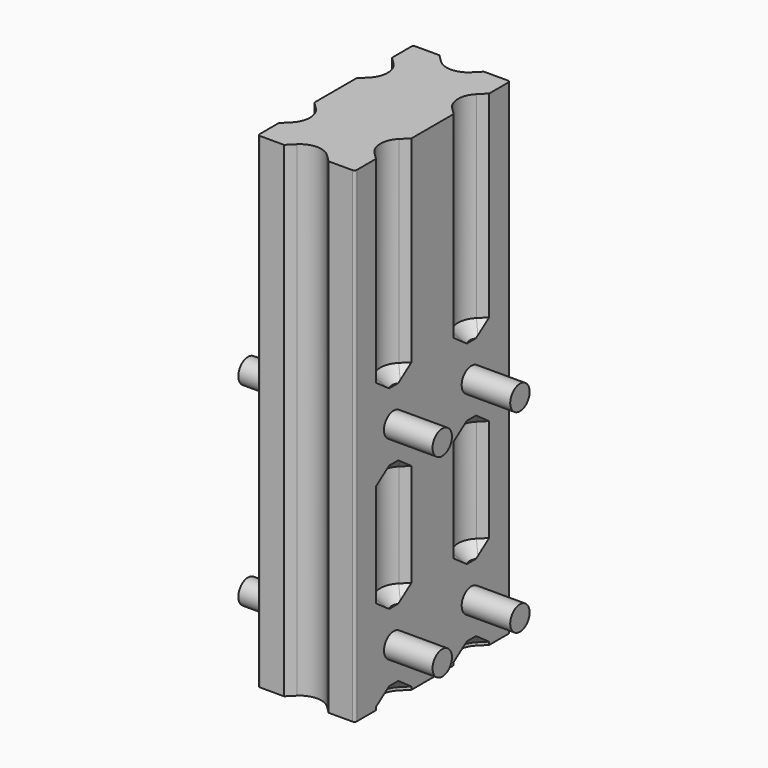
from build123d import *

# Parameters (mm, degrees)
F1_DEPTH      = 100
F2_W          = 14
F2_H          = 14
F2_R          = 2.5
F3_DEPTH      = 10
F4_DEPTH      = 20
F5_T4_ANGLE   = 90
F5_T9_ANGLE   = 90
F5_T14_ANGLE  = 90
F5_T19_ANGLE  = 90
F5_T24_ANGLE  = 90
F5_T29_ANGLE  = 90
F5_T34_ANGLE  = 90
F5_T39_ANGLE  = 90
F5_T44_ANGLE  = 90
F5_T49_ANGLE  = 90
F5_T54_ANGLE  = 90
F5_T59_ANGLE  = 90
F5_T64_ANGLE  = 90
F5_T69_ANGLE  = 90
F5_T74_ANGLE  = 90
F5_T79_ANGLE  = 90
F5_T84_DEPTH  = 8.2297199044
F5_T89_DEPTH  = 8.2297199044
F5_T94_DEPTH  = 8.2297199044
F5_T99_DEPTH  = 8.2297199044
F5_T104_DEPTH = 8.2297199044
F5_T109_DEPTH = 8.2297199044
F5_T114_DEPTH = 8.2297199044
F5_T119_DEPTH = 8.2297199044
F5_T124_DEPTH = 8.2297199044
F5_T129_DEPTH = 8.2297199044
F5_T134_DEPTH = 8.2297199044
F5_T139_DEPTH = 8.2297199044
F5_T144_DEPTH = 8.2297199044
F5_T149_DEPTH = 8.2297199044
F5_T154_DEPTH = 8.2297199044
F5_T159_DEPTH = 8.2297199044
F5_T164_DEPTH = 8.2297199044
F5_T169_DEPTH = 8.2297199044
F5_T174_DEPTH = 8.2297199044
F5_T179_DEPTH = 8.2297199044
F5_T184_DEPTH = 8.2297199044
F5_T189_DEPTH = 8.2297199044
F5_T194_DEPTH = 8.2297199044
F5_T199_DEPTH = 8.2297199044
F5_T204_DEPTH = 8.2297199044
F5_T209_DEPTH = 8.2297199044
F5_T214_DEPTH = 8.2297199044
F5_T219_DEPTH = 8.2297199044
F5_T224_DEPTH = 8.2297199044
F5_T229_DEPTH = 8.2297199044
F5_T234_DEPTH = 8.2297199044
F5_T239_DEPTH = 8.2297199044


# Not quite as in the source:
# - a fillet or chamfer that OpenCascade refuses, or shapes differently, is made with other operations: its cross-section is extruded or revolved along the edge and cut away or added


with BuildPart() as f1:
    # F0 (on Top) → F1 (new body)
    with BuildSketch(Plane.XY):
        with BuildLine():
            Line((-10, 5.42), (-10, 0))
            Line((-10, 0), (-10, -5.42))
            Line((-10, -5.42), (-8.545, -6.875))
            Line((-8.545, -6.875), (-8.2, -6.875))
            Line((-8.2, -6.875), (-6.2, -6.875))
            Line((-6.2, -6.875), (-6.2, -13.125))
            Line((-6.2, -13.125), (-8.2, -13.125))
            Line((-8.2, -13.125), (-8.545, -13.125))
            Line((-8.545, -13.125), (-10, -14.58))
            Line((-10, -14.58), (-10, -19.5))
            ThreePointArc((-10, -19.5), (-9.8535533906, -19.8535533906), (-9.5, -20))
            Line((-9.5, -20), (-4.58, -20))
            Line((-4.58, -20), (-3.125, -18.545))
            Line((-3.125, -18.545), (-3.125, -18.2))
            Line((-3.125, -18.2), (-3.125, -16.2))
            Line((-3.125, -16.2), (0, -16.2))
            Line((0, -16.2), (3.125, -16.2))
            Line((3.125, -16.2), (3.125, -18.2))
            Line((3.125, -18.2), (3.125, -18.545))
            Line((3.125, -18.545), (4.58, -20))
            Line((4.58, -20), (9.5, -20))
            ThreePointArc((9.5, -20), (9.8535533906, -19.8535533906), (10, -19.5))
            Line((10, -19.5), (10, -14.58))
            Line((10, -14.58), (8.545, -13.125))
            Line((8.545, -13.125), (8.2, -13.125))
            Line((8.2, -13.125), (6.2, -13.125))
            Line((6.2, -13.125), (6.2, -6.875))
            Line((6.2, -6.875), (8.2, -6.875))
            Line((8.2, -6.875), (8.545, -6.875))
            Line((8.545, -6.875), (10, -5.42))
            Line((10, -5.42), (10, 0))
            Line((10, 0), (10, 5.42))
            Line((10, 5.42), (8.545, 6.875))
            Line((8.545, 6.875), (8.2, 6.875))
            Line((8.2, 6.875), (6.2, 6.875))
            Line((6.2, 6.875), (6.2, 13.125))
            Line((6.2, 13.125), (8.2, 13.125))
            Line((8.2, 13.125), (8.545, 13.125))
            Line((8.545, 13.125), (10, 14.58))
            Line((10, 14.58), (10, 19.5))
            ThreePointArc((10, 19.5), (9.8535533906, 19.8535533906), (9.5, 20))
            Line((9.5, 20), (4.58, 20))
            Line((4.58, 20), (3.125, 18.545))
            Line((3.125, 18.545), (3.125, 18.2))
            Line((3.125, 18.2), (3.125, 16.2))
            Line((3.125, 16.2), (0, 16.2))
            Line((0, 16.2), (-3.125, 16.2))
            Line((-3.125, 16.2), (-3.125, 18.2))
            Line((-3.125, 18.2), (-3.125, 18.545))
            Line((-3.125, 18.545), (-4.58, 20))
            Line((-4.58, 20), (-9.5, 20))
            ThreePointArc((-9.5, 20), (-9.8535533906, 19.8535533906), (-10, 19.5))
            Line((-10, 19.5), (-10, 14.58))
            Line((-10, 14.58), (-8.545, 13.125))
            Line((-8.545, 13.125), (-8.2, 13.125))
            Line((-8.2, 13.125), (-6.2, 13.125))
            Line((-6.2, 13.125), (-6.2, 6.875))
            Line((-6.2, 6.875), (-8.2, 6.875))
            Line((-8.2, 6.875), (-8.545, 6.875))
            Line((-8.545, 6.875), (-10, 5.42))
        make_face()
        with BuildLine():
            ThreePointArc((8.545, 6.875), (7.2505826176, 10), (8.545, 13.125))
            Line((8.545, 13.125), (8.2, 13.125))
            Line((8.2, 13.125), (6.2, 13.125))
            Line((6.2, 13.125), (6.2, 6.875))
            Line((6.2, 6.875), (8.2, 6.875))
            Line((8.2, 6.875), (8.545, 6.875))
        make_face()
        with BuildLine():
            Line((8.2, -13.125), (8.545, -13.125))
            ThreePointArc((8.545, -13.125), (7.2505826176, -10), (8.545, -6.875))
            Line((8.545, -6.875), (8.2, -6.875))
            Line((8.2, -6.875), (6.2, -6.875))
            Line((6.2, -6.875), (6.2, -13.125))
            Line((6.2, -13.125), (8.2, -13.125))
        make_face()
        with BuildLine():
            Line((-3.125, -18.2), (-3.125, -18.545))
            ThreePointArc((-3.125, -18.545), (0, -17.2505826176), (3.125, -18.545))
            Line((3.125, -18.545), (3.125, -18.2))
            Line((3.125, -18.2), (3.125, -16.2))
            Line((3.125, -16.2), (0, -16.2))
            Line((0, -16.2), (-3.125, -16.2))
            Line((-3.125, -16.2), (-3.125, -18.2))
        make_face()
        with BuildLine():
            Line((-8.2, -6.875), (-8.545, -6.875))
            ThreePointArc((-8.545, -6.875), (-7.2505826176, -10), (-8.545, -13.125))
            Line((-8.545, -13.125), (-8.2, -13.125))
            Line((-8.2, -13.125), (-6.2, -13.125))
            Line((-6.2, -13.125), (-6.2, -6.875))
            Line((-6.2, -6.875), (-8.2, -6.875))
        make_face()
        with BuildLine():
            ThreePointArc((-8.545, 13.125), (-7.2505826176, 10), (-8.545, 6.875))
            Line((-8.545, 6.875), (-8.2, 6.875))
            Line((-8.2, 6.875), (-6.2, 6.875))
            Line((-6.2, 6.875), (-6.2, 13.125))
            Line((-6.2, 13.125), (-8.2, 13.125))
            Line((-8.2, 13.125), (-8.545, 13.125))
        make_face()
        with BuildLine():
            ThreePointArc((3.125, 18.545), (0, 17.2505826176), (-3.125, 18.545))
            Line((-3.125, 18.545), (-3.125, 18.2))
            Line((-3.125, 18.2), (-3.125, 16.2))
            Line((-3.125, 16.2), (0, 16.2))
            Line((0, 16.2), (3.125, 16.2))
            Line((3.125, 16.2), (3.125, 18.2))
            Line((3.125, 18.2), (3.125, 18.545))
        make_face()
    extrude(amount=F1_DEPTH)

    # F2 (on Right) → F3 (join, symmetric)
    with BuildSketch(Plane.YZ):
        with Locations((10, 50)):
            Rectangle(F2_W, F2_H)
        with Locations((10, 50)):
            Circle(F2_R, mode=Mode.SUBTRACT)
        with Locations((-10, 50)):
            Rectangle(F2_W, F2_H)
        with Locations((-10, 50)):
            Circle(F2_R, mode=Mode.SUBTRACT)
        with Locations((-10, 10)):
            Rectangle(F2_W, F2_H)
        with Locations((-10, 10)):
            Circle(F2_R, mode=Mode.SUBTRACT)
        with Locations((10, 10)):
            Rectangle(F2_W, F2_H)
        with Locations((10, 10)):
            Circle(F2_R, mode=Mode.SUBTRACT)
    extrude(amount=F3_DEPTH, both=True)

    # F2 (on Right) → F4 (join, symmetric)
    with BuildSketch(Plane.YZ):
        with Locations((10, 10)):
            Circle(F2_R)
        with Locations((10, 50)):
            Circle(F2_R)
        with Locations((-10, 10)):
            Circle(F2_R)
        with Locations((-10, 50)):
            Circle(F2_R)
    extrude(amount=F4_DEPTH, both=True)

    # F5: chamfer of 2.4 on 48 edges, made by hand


with BuildPart() as f5_tool2:
    # F5_s3 → F5_t4 (revolve)
    with BuildSketch(Plane(origin=(-10.835, 10.835, 0), x_dir=(0, 0, 1), z_dir=(-0.7071067812, 0.7071067812, 0))):
        Polygon((43, 0.8385490578), (40.6, 3.2385490578), (43, 3.2385490578), align=None)
    revolve(axis=Axis((-11.67, 10, 43), (0, 0, -1)), revolution_arc=F5_T4_ANGLE)

    split(bisect_by=Plane.YZ.offset(-10), keep=Keep.TOP)


with BuildPart() as f1_1:
    add(f1.part)

    # F5_t1: union F5_tool2
    add(f5_tool2.part)


with BuildPart() as f5_tool7:
    # F5_s8 → F5_t9 (revolve)
    with BuildSketch(Plane(origin=(-10.835, 10.835, 0), x_dir=(0, 0, 1), z_dir=(-0.7071067812, 0.7071067812, 0))):
        Polygon((17, 0.8385490578), (19.4, 3.2385490578), (17, 3.2385490578), align=None)
    revolve(axis=Axis((-11.67, 10, 17), (0, 0, -1)), revolution_arc=F5_T9_ANGLE)

    split(bisect_by=Plane.YZ.offset(-10), keep=Keep.TOP)


with BuildPart() as f1_2:
    add(f1_1.part)

    # F5_t6: union F5_tool7
    add(f5_tool7.part)


with BuildPart() as f5_tool12:
    # F5_s13 → F5_t14 (revolve)
    with BuildSketch(Plane(origin=(-10.835, 10.835, 0), x_dir=(0, 0, 1), z_dir=(-0.7071067812, 0.7071067812, 0))):
        Polygon((57, 0.8385490578), (59.4, 3.2385490578), (57, 3.2385490578), align=None)
    revolve(axis=Axis((-11.67, 10, 57), (0, 0, -1)), revolution_arc=F5_T14_ANGLE)

    split(bisect_by=Plane.YZ.offset(-10), keep=Keep.TOP)


with BuildPart() as f1_3:
    add(f1_2.part)

    # F5_t11: union F5_tool12
    add(f5_tool12.part)


with BuildPart() as f5_tool17:
    # F5_s18 → F5_t19 (revolve)
    with BuildSketch(Plane(origin=(-0.835, 0.835, 0), x_dir=(0, 0, 1), z_dir=(-0.7071067812, 0.7071067812, 0))):
        Polygon((57, -13.3035865659), (59.4, -10.9035865659), (57, -10.9035865659), align=None)
    revolve(axis=Axis((-11.67, -10, 57), (0, 0, -1)), revolution_arc=F5_T19_ANGLE)

    split(bisect_by=Plane.YZ.offset(-10), keep=Keep.TOP)


with BuildPart() as f1_4:
    add(f1_3.part)

    # F5_t16: union F5_tool17
    add(f5_tool17.part)


with BuildPart() as f5_tool22:
    # F5_s23 → F5_t24 (revolve)
    with BuildSketch(Plane(origin=(-0.835, 0.835, 0), x_dir=(0, 0, 1), z_dir=(-0.7071067812, 0.7071067812, 0))):
        Polygon((17, -13.3035865659), (19.4, -10.9035865659), (17, -10.9035865659), align=None)
    revolve(axis=Axis((-11.67, -10, 17), (0, 0, -1)), revolution_arc=F5_T24_ANGLE)

    split(bisect_by=Plane.YZ.offset(-10), keep=Keep.TOP)


with BuildPart() as f1_5:
    add(f1_4.part)

    # F5_t21: union F5_tool22
    add(f5_tool22.part)


with BuildPart() as f5_tool27:
    # F5_s28 → F5_t29 (revolve)
    with BuildSketch(Plane(origin=(-0.835, 0.835, 0), x_dir=(0, 0, 1), z_dir=(-0.7071067812, 0.7071067812, 0))):
        Polygon((43, -13.3035865659), (40.6, -10.9035865659), (43, -10.9035865659), align=None)
    revolve(axis=Axis((-11.67, -10, 43), (0, 0, -1)), revolution_arc=F5_T29_ANGLE)

    split(bisect_by=Plane.YZ.offset(-10), keep=Keep.TOP)


with BuildPart() as f1_6:
    add(f1_5.part)

    # F5_t26: union F5_tool27
    add(f5_tool27.part)


with BuildPart() as f5_tool32:
    # F5_s33 → F5_t34 (revolve)
    with BuildSketch(Plane(origin=(-0.835, 0.835, 0), x_dir=(0, 0, 1), z_dir=(-0.7071067812, 0.7071067812, 0))):
        Polygon((0.6, -10.9035865659), (3, -13.3035865659), (3, -10.9035865659), align=None)
    revolve(axis=Axis((-11.67, -10, 3), (0, 0, -1)), revolution_arc=F5_T34_ANGLE)

    split(bisect_by=Plane.YZ.offset(-10), keep=Keep.TOP)


with BuildPart() as f1_7:
    add(f1_6.part)

    # F5_t31: union F5_tool32
    add(f5_tool32.part)


with BuildPart() as f5_tool37:
    # F5_s38 → F5_t39 (revolve)
    with BuildSketch(Plane(origin=(-10.835, 10.835, 0), x_dir=(0, 0, 1), z_dir=(-0.7071067812, 0.7071067812, 0))):
        Polygon((3, 0.8385490578), (0.6, 3.2385490578), (3, 3.2385490578), align=None)
    revolve(axis=Axis((-11.67, 10, 3), (0, 0, -1)), revolution_arc=F5_T39_ANGLE)

    split(bisect_by=Plane.YZ.offset(-10), keep=Keep.TOP)


with BuildPart() as f1_8:
    add(f1_7.part)

    # F5_t36: union F5_tool37
    add(f5_tool37.part)


with BuildPart() as f5_tool42:
    # F5_s43 → F5_t44 (revolve)
    with BuildSketch(Plane(origin=(10.835, -10.835, 0), x_dir=(0, 0, 1), z_dir=(0.7071067812, -0.7071067812, 0))):
        Polygon((57, 0.8385490578), (59.4, 3.2385490578), (57, 3.2385490578), align=None)
    revolve(axis=Axis((11.67, -10, 57), (0, 0, -1)), revolution_arc=F5_T44_ANGLE)

    split(bisect_by=Plane.YZ.offset(10), keep=Keep.BOTTOM)


with BuildPart() as f1_9:
    add(f1_8.part)

    # F5_t41: union F5_tool42
    add(f5_tool42.part)


with BuildPart() as f5_tool47:
    # F5_s48 → F5_t49 (revolve)
    with BuildSketch(Plane(origin=(10.835, -10.835, 0), x_dir=(0, 0, 1), z_dir=(0.7071067812, -0.7071067812, 0))):
        Polygon((17, 0.8385490578), (19.4, 3.2385490578), (17, 3.2385490578), align=None)
    revolve(axis=Axis((11.67, -10, 17), (0, 0, -1)), revolution_arc=F5_T49_ANGLE)

    split(bisect_by=Plane.YZ.offset(10), keep=Keep.BOTTOM)


with BuildPart() as f1_10:
    add(f1_9.part)

    # F5_t46: union F5_tool47
    add(f5_tool47.part)


with BuildPart() as f5_tool52:
    # F5_s53 → F5_t54 (revolve)
    with BuildSketch(Plane(origin=(0.835, -0.835, 0), x_dir=(0, 0, 1), z_dir=(0.7071067812, -0.7071067812, 0))):
        Polygon((17, -13.3035865659), (19.4, -10.9035865659), (17, -10.9035865659), align=None)
    revolve(axis=Axis((11.67, 10, 17), (0, 0, -1)), revolution_arc=F5_T54_ANGLE)

    split(bisect_by=Plane.YZ.offset(10), keep=Keep.BOTTOM)


with BuildPart() as f1_11:
    add(f1_10.part)

    # F5_t51: union F5_tool52
    add(f5_tool52.part)


with BuildPart() as f5_tool57:
    # F5_s58 → F5_t59 (revolve)
    with BuildSketch(Plane(origin=(0.835, -0.835, 0), x_dir=(0, 0, 1), z_dir=(0.7071067812, -0.7071067812, 0))):
        Polygon((57, -13.3035865659), (59.4, -10.9035865659), (57, -10.9035865659), align=None)
    revolve(axis=Axis((11.67, 10, 57), (0, 0, -1)), revolution_arc=F5_T59_ANGLE)

    split(bisect_by=Plane.YZ.offset(10), keep=Keep.BOTTOM)


with BuildPart() as f1_12:
    add(f1_11.part)

    # F5_t56: union F5_tool57
    add(f5_tool57.part)


with BuildPart() as f5_tool62:
    # F5_s63 → F5_t64 (revolve)
    with BuildSketch(Plane(origin=(0.835, -0.835, 0), x_dir=(0, 0, 1), z_dir=(0.7071067812, -0.7071067812, 0))):
        Polygon((43, -13.3035865659), (40.6, -10.9035865659), (43, -10.9035865659), align=None)
    revolve(axis=Axis((11.67, 10, 43), (0, 0, -1)), revolution_arc=F5_T64_ANGLE)

    split(bisect_by=Plane.YZ.offset(10), keep=Keep.BOTTOM)


with BuildPart() as f1_13:
    add(f1_12.part)

    # F5_t61: union F5_tool62
    add(f5_tool62.part)


with BuildPart() as f5_tool67:
    # F5_s68 → F5_t69 (revolve)
    with BuildSketch(Plane(origin=(10.835, -10.835, 0), x_dir=(0, 0, 1), z_dir=(0.7071067812, -0.7071067812, 0))):
        Polygon((43, 0.8385490578), (40.6, 3.2385490578), (43, 3.2385490578), align=None)
    revolve(axis=Axis((11.67, -10, 43), (0, 0, -1)), revolution_arc=F5_T69_ANGLE)

    split(bisect_by=Plane.YZ.offset(10), keep=Keep.BOTTOM)


with BuildPart() as f1_14:
    add(f1_13.part)

    # F5_t66: union F5_tool67
    add(f5_tool67.part)


with BuildPart() as f5_tool72:
    # F5_s73 → F5_t74 (revolve)
    with BuildSketch(Plane(origin=(10.835, -10.835, 0), x_dir=(0, 0, 1), z_dir=(0.7071067812, -0.7071067812, 0))):
        Polygon((0.6, 3.2385490578), (3, 0.8385490578), (3, 3.2385490578), align=None)
    revolve(axis=Axis((11.67, -10, 3), (0, 0, -1)), revolution_arc=F5_T74_ANGLE)

    split(bisect_by=Plane.YZ.offset(10), keep=Keep.BOTTOM)


with BuildPart() as f1_15:
    add(f1_14.part)

    # F5_t71: union F5_tool72
    add(f5_tool72.part)


with BuildPart() as f5_tool77:
    # F5_s78 → F5_t79 (revolve)
    with BuildSketch(Plane(origin=(0.835, -0.835, 0), x_dir=(0, 0, 1), z_dir=(0.7071067812, -0.7071067812, 0))):
        Polygon((0.6, -10.9035865659), (3, -13.3035865659), (3, -10.9035865659), align=None)
    revolve(axis=Axis((11.67, 10, 3), (0, 0, -1)), revolution_arc=F5_T79_ANGLE)

    split(bisect_by=Plane.YZ.offset(10), keep=Keep.BOTTOM)


with BuildPart() as f1_16:
    add(f1_15.part)

    # F5_t76: union F5_tool77
    add(f5_tool77.part)


with BuildPart() as f5_tool82:
    # F5_s83 → F5_t84 (new body)
    with BuildSketch(Plane(origin=(-6.6542907516, -6.6542907516, 0), x_dir=(0, 0, 1), z_dir=(0.7071067812, 0.7071067812, 0))):
        Polygon((0.6, -10.9035865659), (3, -13.3035865659), (3, -10.9035865659), align=None)
    extrude(amount=F5_T84_DEPTH)

    split(bisect_by=Plane.YZ.offset(-10), keep=Keep.TOP)


with BuildPart() as f1_17:
    add(f1_16.part)

    # F5_t81: union F5_tool82
    add(f5_tool82.part)


with BuildPart() as f5_tool87:
    # F5_s88 → F5_t89 (new body)
    with BuildSketch(Plane(origin=(-10.835, 10.835, 0), x_dir=(0, 0, 1), z_dir=(-0.7071067812, 0.7071067812, 0))):
        Polygon((3, 0.8385490578), (0.6, 3.2385490578), (3, 3.2385490578), align=None)
    extrude(amount=F5_T89_DEPTH)

    split(bisect_by=Plane.YZ.offset(-10), keep=Keep.TOP)


with BuildPart() as f1_18:
    add(f1_17.part)

    # F5_t86: union F5_tool87
    add(f5_tool87.part)


with BuildPart() as f5_tool92:
    # F5_s93 → F5_t94 (new body)
    with BuildSketch(Plane(origin=(-0.835, 0.835, 0), x_dir=(0, 0, 1), z_dir=(-0.7071067812, 0.7071067812, 0))):
        Polygon((0.6, -10.9035865659), (3, -13.3035865659), (3, -10.9035865659), align=None)
    extrude(amount=F5_T94_DEPTH)

    split(bisect_by=Plane.YZ.offset(-10), keep=Keep.TOP)


with BuildPart() as f1_19:
    add(f1_18.part)

    # F5_t91: union F5_tool92
    add(f5_tool92.part)


with BuildPart() as f5_tool97:
    # F5_s98 → F5_t99 (new body)
    with BuildSketch(Plane(origin=(-16.6542907516, -16.6542907516, 0), x_dir=(0, 0, 1), z_dir=(0.7071067812, 0.7071067812, 0))):
        Polygon((0.6, 3.2385490578), (3, 0.8385490578), (3, 3.2385490578), align=None)
    extrude(amount=F5_T99_DEPTH)

    split(bisect_by=Plane.YZ.offset(-10), keep=Keep.TOP)


with BuildPart() as f1_20:
    add(f1_19.part)

    # F5_t96: union F5_tool97
    add(f5_tool97.part)


with BuildPart() as f5_tool102:
    # F5_s103 → F5_t104 (new body)
    with BuildSketch(Plane(origin=(10.835, -10.835, 0), x_dir=(0, 0, 1), z_dir=(0.7071067812, -0.7071067812, 0))):
        Polygon((0.6, 3.2385490578), (3, 0.8385490578), (3, 3.2385490578), align=None)
    extrude(amount=F5_T104_DEPTH)

    split(bisect_by=Plane.YZ.offset(10), keep=Keep.BOTTOM)


with BuildPart() as f1_21:
    add(f1_20.part)

    # F5_t101: union F5_tool102
    add(f5_tool102.part)


with BuildPart() as f5_tool107:
    # F5_s108 → F5_t109 (new body)
    with BuildSketch(Plane(origin=(6.6542907516, 6.6542907516, 0), x_dir=(0, 0, 1), z_dir=(-0.7071067812, -0.7071067812, 0))):
        Polygon((0.6, -10.9035865659), (3, -13.3035865659), (3, -10.9035865659), align=None)
    extrude(amount=F5_T109_DEPTH)

    split(bisect_by=Plane.YZ.offset(10), keep=Keep.BOTTOM)


with BuildPart() as f1_22:
    add(f1_21.part)

    # F5_t106: union F5_tool107
    add(f5_tool107.part)


with BuildPart() as f5_tool112:
    # F5_s113 → F5_t114 (new body)
    with BuildSketch(Plane(origin=(0.835, -0.835, 0), x_dir=(0, 0, 1), z_dir=(0.7071067812, -0.7071067812, 0))):
        Polygon((0.6, -10.9035865659), (3, -13.3035865659), (3, -10.9035865659), align=None)
    extrude(amount=F5_T114_DEPTH)

    split(bisect_by=Plane.YZ.offset(10), keep=Keep.BOTTOM)


with BuildPart() as f1_23:
    add(f1_22.part)

    # F5_t111: union F5_tool112
    add(f5_tool112.part)


with BuildPart() as f5_tool117:
    # F5_s118 → F5_t119 (new body)
    with BuildSketch(Plane(origin=(16.6542907516, 16.6542907516, 0), x_dir=(0, 0, 1), z_dir=(-0.7071067812, -0.7071067812, 0))):
        Polygon((0.6, 3.2385490578), (3, 0.8385490578), (3, 3.2385490578), align=None)
    extrude(amount=F5_T119_DEPTH)

    split(bisect_by=Plane.YZ.offset(10), keep=Keep.BOTTOM)


with BuildPart() as f1_24:
    add(f1_23.part)

    # F5_t116: union F5_tool117
    add(f5_tool117.part)


with BuildPart() as f5_tool122:
    # F5_s123 → F5_t124 (new body)
    with BuildSketch(Plane(origin=(-16.6542907516, 16.6542907516, 0), x_dir=(0, 0, 1), z_dir=(0.7071067812, -0.7071067812, 0))):
        Polygon((59.4, -3.2385490578), (57, -0.8385490578), (57, -3.2385490578), align=None)
    extrude(amount=F5_T124_DEPTH)

    split(bisect_by=Plane.YZ.offset(-10), keep=Keep.TOP)


with BuildPart() as f1_25:
    add(f1_24.part)

    # F5_t121: union F5_tool122
    add(f5_tool122.part)


with BuildPart() as f5_tool127:
    # F5_s128 → F5_t129 (new body)
    with BuildSketch(Plane(origin=(-0.835, -0.835, 0), x_dir=(0, 0, 1), z_dir=(-0.7071067812, -0.7071067812, 0))):
        Polygon((57, 13.3035865659), (59.4, 10.9035865659), (57, 10.9035865659), align=None)
    extrude(amount=F5_T129_DEPTH)

    split(bisect_by=Plane.YZ.offset(-10), keep=Keep.TOP)


with BuildPart() as f1_26:
    add(f1_25.part)

    # F5_t126: union F5_tool127
    add(f5_tool127.part)


with BuildPart() as f5_tool132:
    # F5_s133 → F5_t134 (new body)
    with BuildSketch(Plane(origin=(-6.6542907516, 6.6542907516, 0), x_dir=(0, 0, 1), z_dir=(0.7071067812, -0.7071067812, 0))):
        Polygon((59.4, 10.9035865659), (57, 13.3035865659), (57, 10.9035865659), align=None)
    extrude(amount=F5_T134_DEPTH)

    split(bisect_by=Plane.YZ.offset(-10), keep=Keep.TOP)


with BuildPart() as f1_27:
    add(f1_26.part)

    # F5_t131: union F5_tool132
    add(f5_tool132.part)


with BuildPart() as f5_tool137:
    # F5_s138 → F5_t139 (new body)
    with BuildSketch(Plane(origin=(-10.835, -10.835, 0), x_dir=(0, 0, 1), z_dir=(-0.7071067812, -0.7071067812, 0))):
        Polygon((57, -0.8385490578), (59.4, -3.2385490578), (57, -3.2385490578), align=None)
    extrude(amount=F5_T139_DEPTH)

    split(bisect_by=Plane.YZ.offset(-10), keep=Keep.TOP)


with BuildPart() as f1_28:
    add(f1_27.part)

    # F5_t136: union F5_tool137
    add(f5_tool137.part)


with BuildPart() as f5_tool142:
    # F5_s143 → F5_t144 (new body)
    with BuildSketch(Plane(origin=(-6.6542907516, 6.6542907516, 0), x_dir=(0, 0, 1), z_dir=(0.7071067812, -0.7071067812, 0))):
        Polygon((19.4, 10.9035865659), (17, 13.3035865659), (17, 10.9035865659), align=None)
    extrude(amount=F5_T144_DEPTH)

    split(bisect_by=Plane.YZ.offset(-10), keep=Keep.TOP)


with BuildPart() as f1_29:
    add(f1_28.part)

    # F5_t141: union F5_tool142
    add(f5_tool142.part)


with BuildPart() as f5_tool147:
    # F5_s148 → F5_t149 (new body)
    with BuildSketch(Plane(origin=(-0.835, 0.835, 0), x_dir=(0, 0, 1), z_dir=(-0.7071067812, 0.7071067812, 0))):
        Polygon((40.6, -10.9035865659), (43, -13.3035865659), (43, -10.9035865659), align=None)
    extrude(amount=F5_T149_DEPTH)

    split(bisect_by=Plane.YZ.offset(-10), keep=Keep.TOP)


with BuildPart() as f1_30:
    add(f1_29.part)

    # F5_t146: union F5_tool147
    add(f5_tool147.part)


with BuildPart() as f5_tool152:
    # F5_s153 → F5_t154 (new body)
    with BuildSketch(Plane(origin=(-10.835, -10.835, 0), x_dir=(0, 0, 1), z_dir=(-0.7071067812, -0.7071067812, 0))):
        Polygon((17, -0.8385490578), (19.4, -3.2385490578), (17, -3.2385490578), align=None)
    extrude(amount=F5_T154_DEPTH)

    split(bisect_by=Plane.YZ.offset(-10), keep=Keep.TOP)


with BuildPart() as f1_31:
    add(f1_30.part)

    # F5_t151: union F5_tool152
    add(f5_tool152.part)


with BuildPart() as f5_tool157:
    # F5_s158 → F5_t159 (new body)
    with BuildSketch(Plane(origin=(-16.6542907516, -16.6542907516, 0), x_dir=(0, 0, 1), z_dir=(0.7071067812, 0.7071067812, 0))):
        Polygon((40.6, 3.2385490578), (43, 0.8385490578), (43, 3.2385490578), align=None)
    extrude(amount=F5_T159_DEPTH)

    split(bisect_by=Plane.YZ.offset(-10), keep=Keep.TOP)


with BuildPart() as f1_32:
    add(f1_31.part)

    # F5_t156: union F5_tool157
    add(f5_tool157.part)


with BuildPart() as f5_tool162:
    # F5_s163 → F5_t164 (new body)
    with BuildSketch(Plane(origin=(-0.835, -0.835, 0), x_dir=(0, 0, 1), z_dir=(-0.7071067812, -0.7071067812, 0))):
        Polygon((19.4, 10.9035865659), (17, 13.3035865659), (17, 10.9035865659), align=None)
    extrude(amount=F5_T164_DEPTH)

    split(bisect_by=Plane.YZ.offset(-10), keep=Keep.TOP)


with BuildPart() as f1_33:
    add(f1_32.part)

    # F5_t161: union F5_tool162
    add(f5_tool162.part)


with BuildPart() as f5_tool167:
    # F5_s168 → F5_t169 (new body)
    with BuildSketch(Plane(origin=(-6.6542907516, -6.6542907516, 0), x_dir=(0, 0, 1), z_dir=(0.7071067812, 0.7071067812, 0))):
        Polygon((40.6, -10.9035865659), (43, -13.3035865659), (43, -10.9035865659), align=None)
    extrude(amount=F5_T169_DEPTH)

    split(bisect_by=Plane.YZ.offset(-10), keep=Keep.TOP)


with BuildPart() as f1_34:
    add(f1_33.part)

    # F5_t166: union F5_tool167
    add(f5_tool167.part)


with BuildPart() as f5_tool172:
    # F5_s173 → F5_t174 (new body)
    with BuildSketch(Plane(origin=(-10.835, 10.835, 0), x_dir=(0, 0, 1), z_dir=(-0.7071067812, 0.7071067812, 0))):
        Polygon((43, 0.8385490578), (40.6, 3.2385490578), (43, 3.2385490578), align=None)
    extrude(amount=F5_T174_DEPTH)

    split(bisect_by=Plane.YZ.offset(-10), keep=Keep.TOP)


with BuildPart() as f1_35:
    add(f1_34.part)

    # F5_t171: union F5_tool172
    add(f5_tool172.part)


with BuildPart() as f5_tool177:
    # F5_s178 → F5_t179 (new body)
    with BuildSketch(Plane(origin=(-16.6542907516, 16.6542907516, 0), x_dir=(0, 0, 1), z_dir=(0.7071067812, -0.7071067812, 0))):
        Polygon((19.4, -3.2385490578), (17, -0.8385490578), (17, -3.2385490578), align=None)
    extrude(amount=F5_T179_DEPTH)

    split(bisect_by=Plane.YZ.offset(-10), keep=Keep.TOP)


with BuildPart() as f1_36:
    add(f1_35.part)

    # F5_t176: union F5_tool177
    add(f5_tool177.part)


with BuildPart() as f5_tool182:
    # F5_s183 → F5_t184 (new body)
    with BuildSketch(Plane(origin=(16.6542907516, -16.6542907516, 0), x_dir=(0, 0, 1), z_dir=(-0.7071067812, 0.7071067812, 0))):
        Polygon((59.4, -3.2385490578), (57, -0.8385490578), (57, -3.2385490578), align=None)
    extrude(amount=F5_T184_DEPTH)

    split(bisect_by=Plane.YZ.offset(10), keep=Keep.BOTTOM)


with BuildPart() as f1_37:
    add(f1_36.part)

    # F5_t181: union F5_tool182
    add(f5_tool182.part)


with BuildPart() as f5_tool187:
    # F5_s188 → F5_t189 (new body)
    with BuildSketch(Plane(origin=(0.835, 0.835, 0), x_dir=(0, 0, 1), z_dir=(0.7071067812, 0.7071067812, 0))):
        Polygon((57, 13.3035865659), (59.4, 10.9035865659), (57, 10.9035865659), align=None)
    extrude(amount=F5_T189_DEPTH)

    split(bisect_by=Plane.YZ.offset(10), keep=Keep.BOTTOM)


with BuildPart() as f1_38:
    add(f1_37.part)

    # F5_t186: union F5_tool187
    add(f5_tool187.part)


with BuildPart() as f5_tool192:
    # F5_s193 → F5_t194 (new body)
    with BuildSketch(Plane(origin=(6.6542907516, -6.6542907516, 0), x_dir=(0, 0, 1), z_dir=(-0.7071067812, 0.7071067812, 0))):
        Polygon((59.4, 10.9035865659), (57, 13.3035865659), (57, 10.9035865659), align=None)
    extrude(amount=F5_T194_DEPTH)

    split(bisect_by=Plane.YZ.offset(10), keep=Keep.BOTTOM)


with BuildPart() as f1_39:
    add(f1_38.part)

    # F5_t191: union F5_tool192
    add(f5_tool192.part)


with BuildPart() as f5_tool197:
    # F5_s198 → F5_t199 (new body)
    with BuildSketch(Plane(origin=(10.835, 10.835, 0), x_dir=(0, 0, 1), z_dir=(0.7071067812, 0.7071067812, 0))):
        Polygon((57, -0.8385490578), (59.4, -3.2385490578), (57, -3.2385490578), align=None)
    extrude(amount=F5_T199_DEPTH)

    split(bisect_by=Plane.YZ.offset(10), keep=Keep.BOTTOM)


with BuildPart() as f1_40:
    add(f1_39.part)

    # F5_t196: union F5_tool197
    add(f5_tool197.part)


with BuildPart() as f5_tool202:
    # F5_s203 → F5_t204 (new body)
    with BuildSketch(Plane(origin=(16.6542907516, -16.6542907516, 0), x_dir=(0, 0, 1), z_dir=(-0.7071067812, 0.7071067812, 0))):
        Polygon((19.4, -3.2385490578), (17, -0.8385490578), (17, -3.2385490578), align=None)
    extrude(amount=F5_T204_DEPTH)

    split(bisect_by=Plane.YZ.offset(10), keep=Keep.BOTTOM)


with BuildPart() as f1_41:
    add(f1_40.part)

    # F5_t201: union F5_tool202
    add(f5_tool202.part)


with BuildPart() as f5_tool207:
    # F5_s208 → F5_t209 (new body)
    with BuildSketch(Plane(origin=(10.835, -10.835, 0), x_dir=(0, 0, 1), z_dir=(0.7071067812, -0.7071067812, 0))):
        Polygon((40.6, 3.2385490578), (43, 0.8385490578), (43, 3.2385490578), align=None)
    extrude(amount=F5_T209_DEPTH)

    split(bisect_by=Plane.YZ.offset(10), keep=Keep.BOTTOM)


with BuildPart() as f1_42:
    add(f1_41.part)

    # F5_t206: union F5_tool207
    add(f5_tool207.part)


with BuildPart() as f5_tool212:
    # F5_s213 → F5_t214 (new body)
    with BuildSketch(Plane(origin=(0.835, 0.835, 0), x_dir=(0, 0, 1), z_dir=(0.7071067812, 0.7071067812, 0))):
        Polygon((17, 13.3035865659), (19.4, 10.9035865659), (17, 10.9035865659), align=None)
    extrude(amount=F5_T214_DEPTH)

    split(bisect_by=Plane.YZ.offset(10), keep=Keep.BOTTOM)


with BuildPart() as f1_43:
    add(f1_42.part)

    # F5_t211: union F5_tool212
    add(f5_tool212.part)


with BuildPart() as f5_tool217:
    # F5_s218 → F5_t219 (new body)
    with BuildSketch(Plane(origin=(6.6542907516, 6.6542907516, 0), x_dir=(0, 0, 1), z_dir=(-0.7071067812, -0.7071067812, 0))):
        Polygon((40.6, -10.9035865659), (43, -13.3035865659), (43, -10.9035865659), align=None)
    extrude(amount=F5_T219_DEPTH)

    split(bisect_by=Plane.YZ.offset(10), keep=Keep.BOTTOM)


with BuildPart() as f1_44:
    add(f1_43.part)

    # F5_t216: union F5_tool217
    add(f5_tool217.part)


with BuildPart() as f5_tool222:
    # F5_s223 → F5_t224 (new body)
    with BuildSketch(Plane(origin=(6.6542907516, -6.6542907516, 0), x_dir=(0, 0, 1), z_dir=(-0.7071067812, 0.7071067812, 0))):
        Polygon((19.4, 10.9035865659), (17, 13.3035865659), (17, 10.9035865659), align=None)
    extrude(amount=F5_T224_DEPTH)

    split(bisect_by=Plane.YZ.offset(10), keep=Keep.BOTTOM)


with BuildPart() as f1_45:
    add(f1_44.part)

    # F5_t221: union F5_tool222
    add(f5_tool222.part)


with BuildPart() as f5_tool227:
    # F5_s228 → F5_t229 (new body)
    with BuildSketch(Plane(origin=(0.835, -0.835, 0), x_dir=(0, 0, 1), z_dir=(0.7071067812, -0.7071067812, 0))):
        Polygon((40.6, -10.9035865659), (43, -13.3035865659), (43, -10.9035865659), align=None)
    extrude(amount=F5_T229_DEPTH)

    split(bisect_by=Plane.YZ.offset(10), keep=Keep.BOTTOM)


with BuildPart() as f1_46:
    add(f1_45.part)

    # F5_t226: union F5_tool227
    add(f5_tool227.part)


with BuildPart() as f5_tool232:
    # F5_s233 → F5_t234 (new body)
    with BuildSketch(Plane(origin=(10.835, 10.835, 0), x_dir=(0, 0, 1), z_dir=(0.7071067812, 0.7071067812, 0))):
        Polygon((17, -0.8385490578), (19.4, -3.2385490578), (17, -3.2385490578), align=None)
    extrude(amount=F5_T234_DEPTH)

    split(bisect_by=Plane.YZ.offset(10), keep=Keep.BOTTOM)


with BuildPart() as f1_47:
    add(f1_46.part)

    # F5_t231: union F5_tool232
    add(f5_tool232.part)


with BuildPart() as f5_tool237:
    # F5_s238 → F5_t239 (new body)
    with BuildSketch(Plane(origin=(16.6542907516, 16.6542907516, 0), x_dir=(0, 0, 1), z_dir=(-0.7071067812, -0.7071067812, 0))):
        Polygon((40.6, 3.2385490578), (43, 0.8385490578), (43, 3.2385490578), align=None)
    extrude(amount=F5_T239_DEPTH)

    split(bisect_by=Plane.YZ.offset(10), keep=Keep.BOTTOM)


with BuildPart() as f1_48:
    add(f1_47.part)

    # F5_t236: union F5_tool237
    add(f5_tool237.part)


solid = f1_48.part
